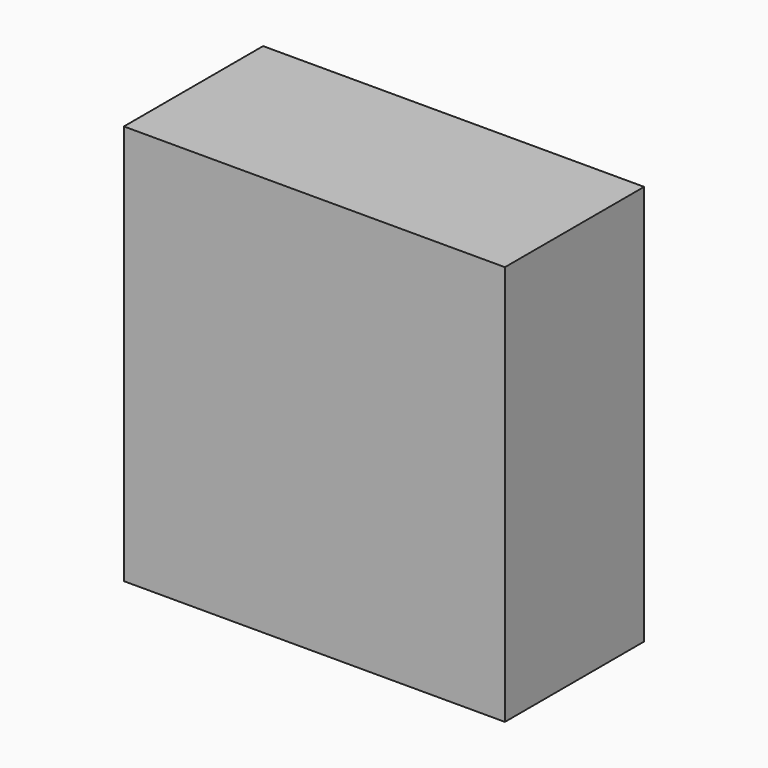
from build123d import *

# Parameters (mm, degrees)
F0_W     = 54.7410696745
F0_H     = 57.5148873031
F1_DEPTH = 25


# Not quite as in the source:
# - the program builds the solid bodies; features that only make, move or delete a surface that nothing else refers to are left out


with BuildPart() as f1:
    # F0 (on Front) → F1 (new body)
    with BuildSketch(Plane.XZ):
        with Locations((-103.307120502, 28.7574436516)):
            Rectangle(F0_W, F0_H)
    extrude(amount=F1_DEPTH)


solid = f1.part
